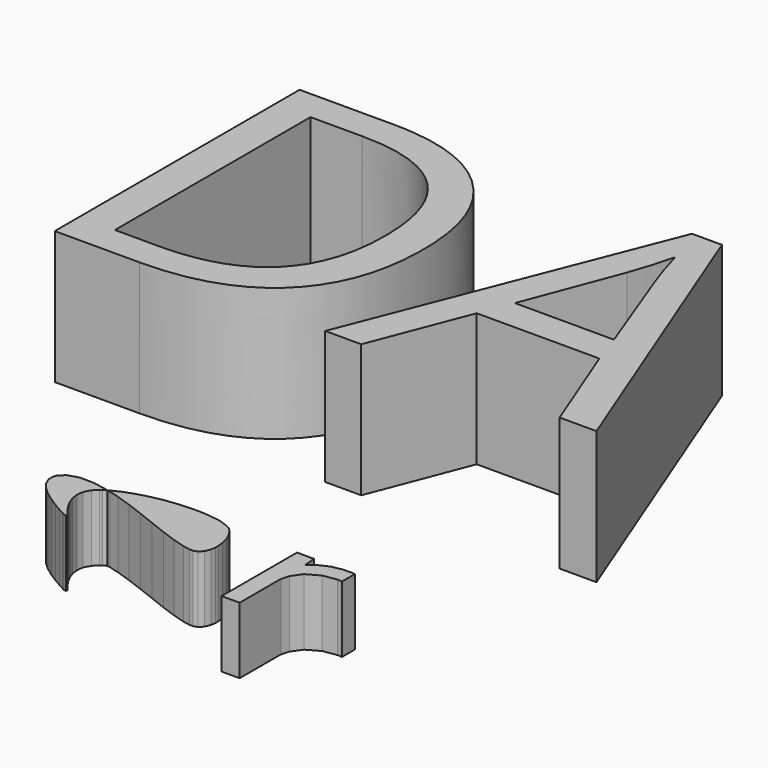
from build123d import *

# Parameters (mm, degrees)
F1_DEPTH     = 12.7
F2_TEXT_SIZE = 81.8710528274
F3_DEPTH     = 25.4


# Not quite as in the source:
# - a feature names something its author has since deleted; it is built from what else it names
# - Text() gives the source's letters only with a copy of the font that has no kerning and outlines rounded to 1/6400 em; it was checked with that copy


with BuildPart() as f1:
    # F0 (on Top) → F1 (new body)
    with BuildSketch(Plane.XY):
        Polygon((37.6745883131, 8.5973698934), (38.5498723131, 8.5475858934), (38.5498723131, 11.5945698934), (37.9623703131, 11.6481638934), (36.1848783131, 11.6169218934), (34.1549103131, 11.2171258934), (32.4117083131, 10.3959438934), (31.2473723131, 9.5013558934), (30.9138703131, 9.1513438934), (30.7348003131, 11.6321618934), (27.4744563131, 11.6321618934), (27.4744563131, -6.3708247066), (30.9138703131, -6.3708247066), (30.9138703131, 2.9570458934), (30.9138703131, 3.4614898934), (31.3273823131, 4.9732978934), (32.6545323131, 6.8457858934), (35.0192723131, 8.1716658934), align=None)
    extrude(amount=F1_DEPTH)


with BuildPart() as f1b:
    # F0 (on Top) → F1, piece 2 (new body)
    with BuildSketch(Plane.XY):
        Polygon((-8.180451, 9.0189558), (-7.856601, 9.2323158), (-7.810119, 9.2640658), (-7.279513, 9.5932498), (-7.226935, 9.6222058), (-7.1666285104, 9.6578084264), (-7.167753, 9.6580198), (-7.1648908296, 9.659698252), (-7.226935, 9.6676718), (-7.969885, 9.8713798), (-10.251567, 10.2739698), (-12.956667, 10.3138478), (-15.037689, 9.6608138), (-16.061563, 8.6067138), (-16.188563, 8.1891378), (-16.276701, 7.9011018), (-16.235045, 6.9407278), (-15.703423, 5.6935878), (-14.720697, 4.4738798), (-13.417169, 3.3052258), (-11.923395, 2.2127718), (-10.364851, 1.2203938), (-8.872347, 0.3522218), (-7.899781, -0.1865122), (-7.574407, -0.3658362), (-7.476363, -0.4194302), (-7.154037, -0.5311902), (-6.905879, -0.5090922), (-6.860413, -0.3272282), (-6.989953, -0.0833882), (-7.047865, -0.0170942), (-7.244969, 0.2102358), (-7.803007, 0.9186418), (-8.546973, 2.0113498), (-9.193403, 3.2127698), (-9.652381, 4.4779438), (-9.835769, 5.7581038), (-9.656445, 7.0093078), (-9.026779, 8.1835498), align=None)
        Polygon((-7.167753, 9.6580198), (-7.1666285104, 9.6578084264), (-7.163689, 9.6595438), (-7.1648908296, 9.659698252), align=None)
        Polygon((-7.163689, 9.6595438), (-7.1666285104, 9.6578084264), (-6.529959, 9.5381318), (-4.643247, 9.0199718), (-1.727073, 8.0458818), (1.414653, 6.8660518), (4.618609, 5.6092598), (7.717663, 4.4075858), (10.548239, 3.3880298), (12.945999, 2.6811478), (14.293977, 2.4164798), (14.744319, 2.4164798), (14.988159, 2.4164798), (15.722727, 2.6712418), (16.415893, 3.3616138), (16.827881, 4.3758358), (16.964533, 5.2981098), (16.964533, 5.6039258), (16.964533, 5.9884818), (16.830675, 7.1375778), (16.437991, 8.6356698), (15.795625, 10.0014278), (15.168753, 10.8817918), (14.916531, 11.1299498), (14.657705, 11.3849658), (13.666597, 11.9318278), (11.882247, 12.4860558), (9.670415, 12.8068578), (7.772781, 12.9102358), (7.140321, 12.9102358), (6.330061, 12.9102358), (3.902075, 12.7710438), (1.050925, 12.4029978), (-1.400937, 11.8822978), (-3.438779, 11.2841278), (-5.049647, 10.6874818), (-6.217031, 10.1665278), (-6.928231, 9.7984818), (-7.1648908296, 9.659698252), align=None)
    extrude(amount=F1_DEPTH)


with BuildPart() as f3:
    # F2 (on Top) → F3 (new body)
    with BuildSketch(Plane.XY):
        with Locations((-58.4034830756, 51.1035351186)):
            Text('DA', F2_TEXT_SIZE, font='Open Sans', text_align=(TextAlign.LEFT, TextAlign.BOTTOM))
    extrude(amount=F3_DEPTH)


solid = Compound([f1.part, f1b.part, f3.part])
